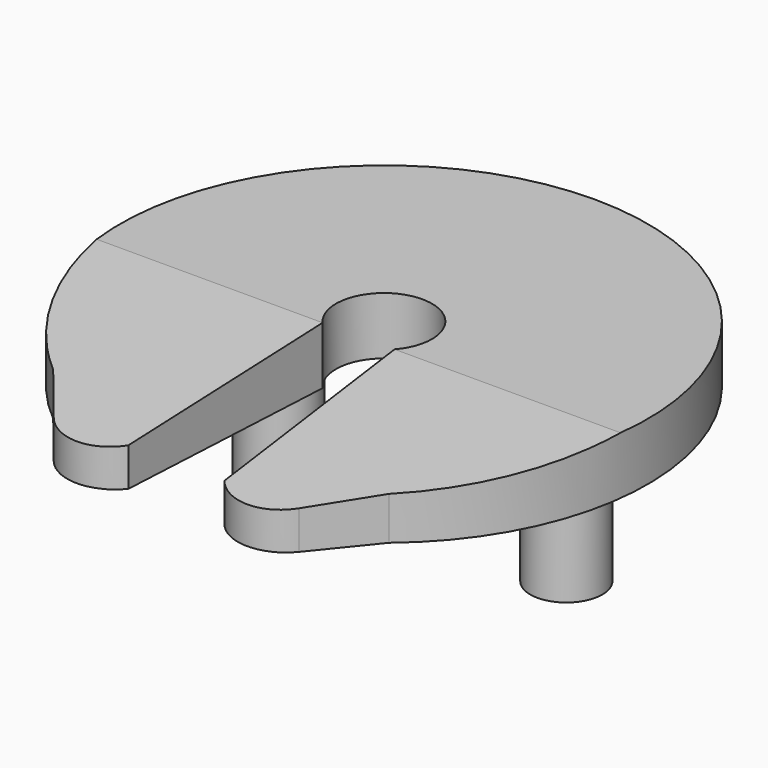
from build123d import *

# Parameters (mm, degrees)
F1_DEPTH = 1.2
F2_R     = 0.75
F3_DEPTH = 3
F7_DEPTH = 18


# Not quite as in the source:
# - an extrude ends at something that could not be found from the text; its depth is read off the source's solid


with BuildPart() as f1:
    # F0 (on Top) → F1 (new body)
    with BuildSketch(Plane.XY):
        with BuildLine():
            ThreePointArc((-0.75, -0.6614378278), (0, 1), (0.75, -0.6614378278))
            Line((0.75, -0.6614378278), (1, -5.4083269132))
            ThreePointArc((1, -5.4083269132), (1.7779895069, -5.7793923244), (2.5559790138, -5.4083269132))
            Line((2.5559790138, -5.4083269132), (3.5, -4.2426406871))
            ThreePointArc((3.5, -4.2426406871), (0, 5.5), (-3.5, -4.2426406871))
            Line((-3.5, -4.2426406871), (-2.5559790138, -5.4083269132))
            ThreePointArc((-2.5559790138, -5.4083269132), (-1.7779895069, -5.7793923244), (-1, -5.4083269132))
            Line((-1, -5.4083269132), (-0.75, -0.6614378278))
        make_face()
    extrude(amount=F1_DEPTH)

    # F2 (on Top) → F3 (join)
    with BuildSketch(Plane.XY):
        with Locations((-3, 1)):
            Circle(F2_R)
        with Locations((3, 1)):
            Circle(F2_R)
    extrude(amount=-F3_DEPTH)

    # F6 (on 3pt) → F7 (cut, through all)
    with BuildSketch(Plane(origin=(0, -0.105069468, 1.2468827773), x_dir=(1, 0, 0), z_dir=(0, -0.0839681251, 0.996468441))):
        Polygon((0.75, -0.558340171), (-0.75, -0.558340171), (-5.460082417, -0.558340171), (-5.460082417, -5.9262430295), (5.460082417, -5.9262430295), (5.460082417, -0.558340171), align=None)
    extrude(amount=F7_DEPTH, mode=Mode.SUBTRACT)


solid = f1.part
